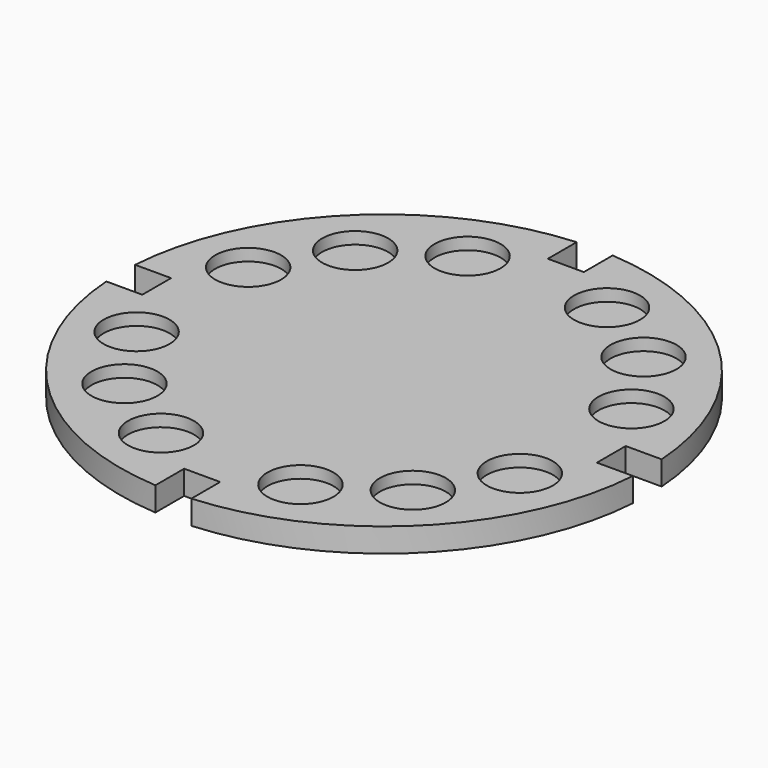
from build123d import *

# Parameters (mm, degrees)
F0_R            = 44.8437
F0_R_2          = 17.4625
F0_W            = 19.05
F0_H            = 6.35
F1_DEPTH        = 12.7
F2_DEPTH        = 6.35
F2_COPIES_COUNT = 4
F3_DEPTH        = 12.701
F3_COPIES_COUNT = 4


# Not quite as in the source:
# - a pattern or mirror of a feature is missing from the dataset's text; its kind, count and spacing are read off the source's solid


with BuildPart() as f1:
    # F0 (on Top) → F1 (new body)
    with BuildSketch(Plane.XY):
        with BuildLine():
            ThreePointArc((-9.525, 139.3749058296), (-95.3557746023, -102.0948884617), (139.7, 0))
            ThreePointArc((139.7, 0), (102.0948884617, 95.3557746023), (9.525, 139.3749058296))
            Line((9.525, 139.3749058296), (9.525, 120.3249058296))
            Line((9.525, 120.3249058296), (9.525, 113.9749058296))
            Line((9.525, 113.9749058296), (-9.525, 113.9749058296))
            Line((-9.525, 113.9749058296), (-9.525, 120.3249058296))
            Line((-9.525, 120.3249058296), (-9.525, 139.3749058296))
        make_face()
        Circle(F0_R, mode=Mode.SUBTRACT)
        with Locations((101.4398184138, 36.921074472)):
            Circle(F0_R_2, mode=Mode.SUBTRACT)
        with Locations((36.921074472, 101.4398184138)):
            Circle(F0_R_2, mode=Mode.SUBTRACT)
        with Locations((76.3321770291, 76.3321770291)):
            Circle(F0_R_2, mode=Mode.SUBTRACT)
        with BuildLine():
            Line((9.525, 120.3249058296), (9.525, 139.3749058296))
            ThreePointArc((9.525, 139.3749058296), (0, 139.7), (-9.525, 139.3749058296))
            Line((-9.525, 139.3749058296), (-9.525, 120.3249058296))
            Line((-9.525, 120.3249058296), (9.525, 120.3249058296))
        make_face()
        with Locations((36.921074472, 101.4398184138)):
            Circle(F0_R_2)
        with Locations((76.3321770291, 76.3321770291)):
            Circle(F0_R_2)
        with Locations((101.4398184138, 36.921074472)):
            Circle(F0_R_2)
        with Locations((0, 117.1499058296)):
            Rectangle(F0_W, F0_H)
        Circle(F0_R)
    extrude(amount=-F1_DEPTH)

    # F0 (on Top) → F2 (cut)
    with BuildSketch(Plane.XY):
        with Locations((36.921074472, 101.4398184138)):
            Circle(F0_R_2)
        with Locations((76.3321770291, 76.3321770291)):
            Circle(F0_R_2)
        with Locations((101.4398184138, 36.921074472)):
            Circle(F0_R_2)
    f2 = extrude(amount=-F2_DEPTH, mode=Mode.SUBTRACT)

    # F2_copies: F2 ×4 about axis
    f2_copies_axis = Axis((0, 0, 0), (0, 0, 1))
    for i in range(1, F2_COPIES_COUNT):
        add(f2.rotate(f2_copies_axis, i * 360 / F2_COPIES_COUNT), mode=Mode.SUBTRACT)

    # F0 (on Top) → F3 (cut, through all)
    with BuildSketch(Plane.XY):
        with BuildLine():
            Line((9.525, 120.3249058296), (9.525, 139.3749058296))
            ThreePointArc((9.525, 139.3749058296), (0, 139.7), (-9.525, 139.3749058296))
            Line((-9.525, 139.3749058296), (-9.525, 120.3249058296))
            Line((-9.525, 120.3249058296), (9.525, 120.3249058296))
        make_face()
    f3 = extrude(amount=-F3_DEPTH, mode=Mode.SUBTRACT)

    # F3_copies: F3 ×4 about axis
    f3_copies_axis = Axis((0, 0, 0), (0, 0, 1))
    for i in range(1, F3_COPIES_COUNT):
        add(f3.rotate(f3_copies_axis, i * 360 / F3_COPIES_COUNT), mode=Mode.SUBTRACT)


solid = f1.part
